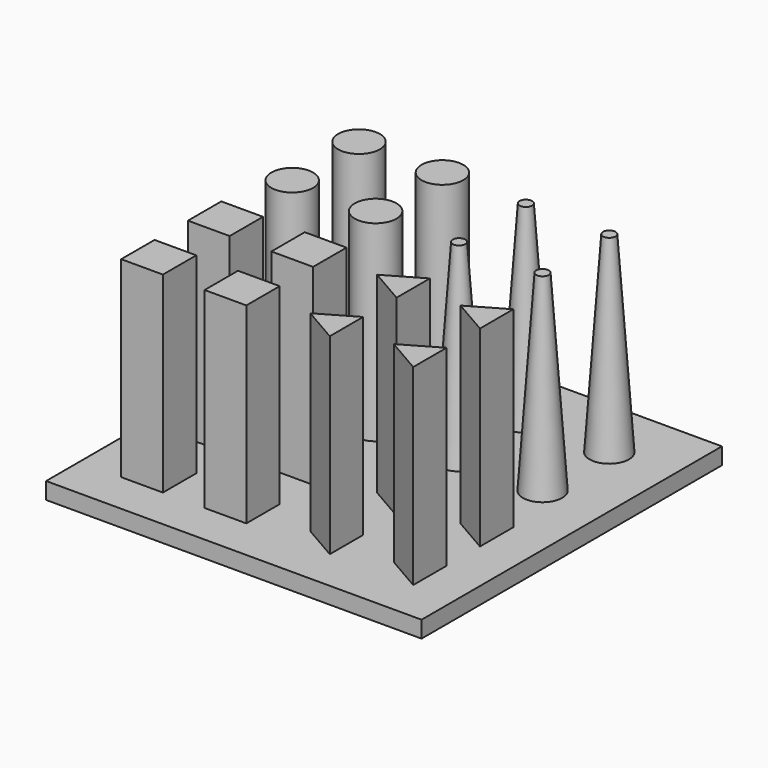
from build123d import *

# Parameters (mm, degrees)
F0_W     = 5
F0_H     = 5
F0_R     = 2.5
F1_DEPTH = 2
F2_DEPTH = 25


# Not quite as in the source:
# - a fillet or chamfer that OpenCascade refuses, or shapes differently, is made with other operations: its cross-section is extruded or revolved along the edge and cut away or added
# - a feature names something its author has since deleted; it is built from what else it names


with BuildPart() as f1:
    # F0 (on Top) → F1 (new body)
    with BuildSketch(Plane.XY):
        Polygon((22.5, 22.5), (-22.5, 22.5), (-22.5, -22.5), (22.5, -22.5), (22.5, -12.5), align=None)
        with Locations((-15, -15)):
            Rectangle(F0_W, F0_H, mode=Mode.SUBTRACT)
        with Locations((-5, -15)):
            Rectangle(F0_W, F0_H, mode=Mode.SUBTRACT)
        with Locations((-15, -5)):
            Rectangle(F0_W, F0_H, mode=Mode.SUBTRACT)
        with Locations((-5, -5)):
            Rectangle(F0_W, F0_H, mode=Mode.SUBTRACT)
        Polygon((7.5, -17.5), (3.1698729811, -15), (7.5, -12.5), align=None, mode=Mode.SUBTRACT)
        Polygon((13.1698729811, -15), (17.5, -12.5), (17.5, -17.5), align=None, mode=Mode.SUBTRACT)
        Polygon((3.1698729811, -5), (7.5, -2.5), (7.5, -7.5), align=None, mode=Mode.SUBTRACT)
        Polygon((17.5, -7.5), (13.1698729811, -5), (17.5, -2.5), align=None, mode=Mode.SUBTRACT)
        with Locations((-15, 5)):
            Circle(F0_R, mode=Mode.SUBTRACT)
        with Locations((-5, 5)):
            Circle(F0_R, mode=Mode.SUBTRACT)
        with Locations((-15, 15)):
            Circle(F0_R, mode=Mode.SUBTRACT)
        with Locations((-5, 15)):
            Circle(F0_R, mode=Mode.SUBTRACT)
        with Locations((5, 5)):
            Circle(F0_R, mode=Mode.SUBTRACT)
        with Locations((15, 5)):
            Circle(F0_R, mode=Mode.SUBTRACT)
        with Locations((5, 15)):
            Circle(F0_R, mode=Mode.SUBTRACT)
        with Locations((15, 15)):
            Circle(F0_R, mode=Mode.SUBTRACT)
    extrude(amount=F1_DEPTH)

    # F0 (on Top) → F2 (join)
    with BuildSketch(Plane.XY):
        with Locations((-15, 15)):
            Circle(F0_R)
        with Locations((-5, 15)):
            Circle(F0_R)
        with Locations((5, 15)):
            Circle(F0_R)
        with Locations((15, 15)):
            Circle(F0_R)
        with Locations((15, 5)):
            Circle(F0_R)
        with Locations((5, 5)):
            Circle(F0_R)
        with Locations((-5, 5)):
            Circle(F0_R)
        with Locations((-15, 5)):
            Circle(F0_R)
        with Locations((-5, -5)):
            Rectangle(F0_W, F0_H)
        with Locations((-15, -5)):
            Rectangle(F0_W, F0_H)
        with Locations((-15, -15)):
            Rectangle(F0_W, F0_H)
        with Locations((-5, -15)):
            Rectangle(F0_W, F0_H)
        Polygon((7.5, -7.5), (7.5, -2.5), (3.1698729811, -5), align=None)
        Polygon((17.5, -2.5), (13.1698729811, -5), (17.5, -7.5), align=None)
        Polygon((7.5, -12.5), (3.1698729811, -15), (7.5, -17.5), align=None)
        Polygon((17.5, -17.5), (17.5, -12.5), (13.1698729811, -15), align=None)
    extrude(amount=F2_DEPTH)

    # F3: chamfer of 25 x 1.7481702986 on 4 edges, made by hand


with BuildPart() as f3_tool2:
    # F3_s3 → F3_t4 (revolve)
    with BuildSketch(Plane.XZ.offset(-15)):
        Polygon((17.5, 0), (15.7518297014, 25), (17.5, 25), align=None)
    revolve(axis=Axis((15, 15, 25), (0, 0, 1)))

    split(bisect_by=Plane.XY.offset(2), keep=Keep.TOP)


with BuildPart() as f1_1:
    add(f1.part)

    # F3_t1: cut F3_tool2
    add(f3_tool2.part, mode=Mode.SUBTRACT)


with BuildPart() as f3_tool7:
    # F3_s8 → F3_t9 (revolve)
    with BuildSketch(Plane.XZ.offset(-5)):
        Polygon((17.5, 0), (15.7518297014, 25), (17.5, 25), align=None)
    revolve(axis=Axis((15, 5, 25), (0, 0, 1)))

    split(bisect_by=Plane.XY.offset(2), keep=Keep.TOP)


with BuildPart() as f1_2:
    add(f1_1.part)

    # F3_t6: cut F3_tool7
    add(f3_tool7.part, mode=Mode.SUBTRACT)


with BuildPart() as f3_tool12:
    # F3_s13 → F3_t14 (revolve)
    with BuildSketch(Plane.XZ.offset(-5)):
        Polygon((7.5, 0), (5.7518297014, 25), (7.5, 25), align=None)
    revolve(axis=Axis((5, 5, 25), (0, 0, 1)))

    split(bisect_by=Plane.XY.offset(2), keep=Keep.TOP)


with BuildPart() as f1_3:
    add(f1_2.part)

    # F3_t11: cut F3_tool12
    add(f3_tool12.part, mode=Mode.SUBTRACT)


with BuildPart() as f3_tool17:
    # F3_s18 → F3_t19 (revolve)
    with BuildSketch(Plane.XZ.offset(-15)):
        Polygon((7.5, 0), (5.7518297014, 25), (7.5, 25), align=None)
    revolve(axis=Axis((5, 15, 25), (0, 0, 1)))

    split(bisect_by=Plane.XY.offset(2), keep=Keep.TOP)


with BuildPart() as f1_4:
    add(f1_3.part)

    # F3_t16: cut F3_tool17
    add(f3_tool17.part, mode=Mode.SUBTRACT)


solid = f1_4.part
